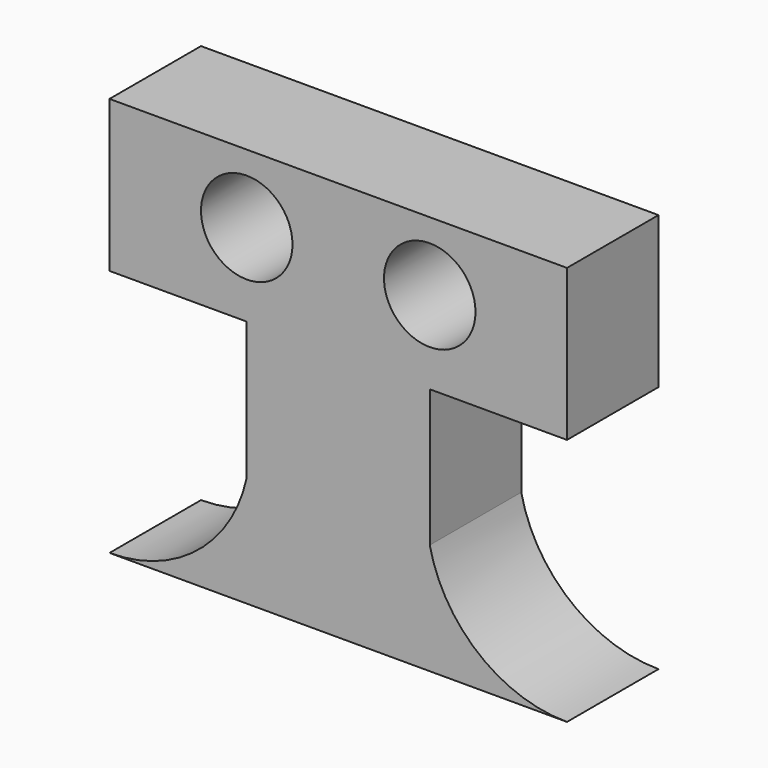
from build123d import *

# Parameters (mm, degrees)
F0_R     = 10
F1_DEPTH = 25


# Not quite as in the source:
# - the program builds the solid bodies; features that only make, move or delete a surface that nothing else refers to are left out


with BuildPart() as f1:
    # F0 (on Front) → F1 (new body)
    with BuildSketch(Plane.XZ):
        with BuildLine():
            ThreePointArc((-20, -21.8138062528), (-30.7082507277, -39.2518025849), (-50, -46.0766659346))
            Line((-50, -46.0766659346), (50, -46.0766659346))
            ThreePointArc((50, -46.0766659346), (30.7082507277, -39.2518025849), (20, -21.8138062528))
            Line((20, -21.8138062528), (20, 8.1861937472))
            Line((20, 8.1861937472), (50, 8.1861937472))
            Line((50, 8.1861937472), (50, 41.2879567593))
            Line((50, 41.2879567593), (-50, 41.2879567593))
            Line((-50, 41.2879567593), (-50, 8.1861937472))
            Line((-50, 8.1861937472), (-20, 8.1861937472))
            Line((-20, 8.1861937472), (-20, -21.8138062528))
        make_face()
        with Locations((-20, 26.2879567593)):
            Circle(F0_R, mode=Mode.SUBTRACT)
        with Locations((20, 26.2879567593)):
            Circle(F0_R, mode=Mode.SUBTRACT)
    extrude(amount=F1_DEPTH)


solid = f1.part
